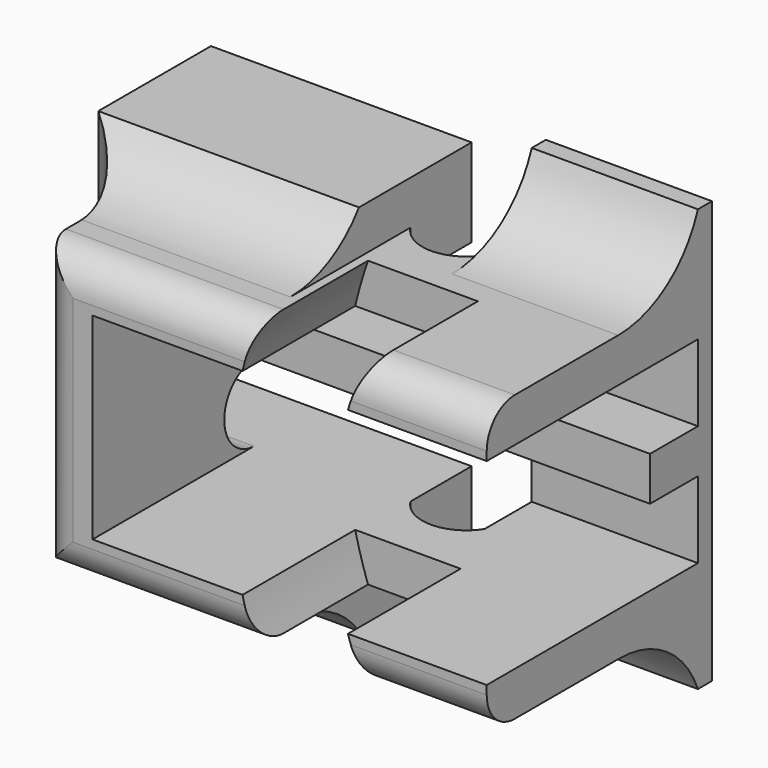
from build123d import *

# Parameters (mm, degrees)
F1_DEPTH      = 2.2
F2_DEPTH      = 4
F3_DEPTH      = 8
F5_W          = 4.721
F5_H          = 0.5
F6_DEPTH      = 2
F6_DEPTH_BACK = 10
F7_DEPTH      = 4
F8_T1_DEPTH   = 5.9270831351
F8_T3_DEPTH   = 8.1
F8_T5_DEPTH   = 4.721
F8_T11_DEPTH  = 12.0188296006
F8_T16_DEPTH  = 14.5648341529
F8_T24_DEPTH  = 14.5648341529
F8_T29_DEPTH  = 12.0188296006
F10_DEPTH     = 1.5
F12_DEPTH     = 2
F13_R         = 1


# Not quite as in the source:
# - a fillet or chamfer that OpenCascade refuses, or shapes differently, is made with other operations: its cross-section is extruded or revolved along the edge and cut away or added


with BuildPart() as f1:
    # F0 (on Front) → F1 (new body)
    with BuildSketch(Plane.XZ):
        with BuildLine():
            Line((-1.6440981598, 0.625), (-5.6, 0.625))
            Line((-5.6, 0.625), (-5.6, -0.625))
            Line((-5.6, -0.625), (-1.6440981598, -0.625))
            ThreePointArc((-1.6440981598, -0.625), (-1.6599999508, 0), (-1.6440981598, 0.625))
        make_face()
        with BuildLine():
            Line((-1.23, 0.625), (-1.6440981598, 0.625))
            ThreePointArc((-1.6440981598, 0.625), (-1.6599999508, 0), (-1.6440981598, -0.625))
            Line((-1.6440981598, -0.625), (-1.23, -0.625))
            Line((-1.23, -0.625), (1.2508001143, -0.625))
            ThreePointArc((1.2508001143, -0.625), (1.23, 0), (1.2508001143, 0.625))
            Line((1.2508001143, 0.625), (-1.23, 0.625))
        make_face()
        with BuildLine():
            Line((1.6420518568, 0.625), (1.2508001143, 0.625))
            ThreePointArc((1.2508001143, 0.625), (1.23, 0), (1.2508001143, -0.625))
            Line((1.2508001143, -0.625), (1.6420518568, -0.625))
            Line((1.6420518568, -0.625), (5.6, -0.625))
            Line((5.6, -0.625), (5.6, 0.625))
            Line((5.6, 0.625), (1.6420518568, 0.625))
        make_face()
    extrude(amount=F1_DEPTH)

    # F0 (on Front) → F2 (join)
    with BuildSketch(Plane.XZ):
        with BuildLine():
            Line((5.6, -2.8), (1.6566885771, -2.8))
            ThreePointArc((1.6566885771, -2.8), (1.8795878526, -3.4337692421), (2.1471830551, -4.05))
            Line((2.1471830551, -4.05), (5.6, -4.05))
            Line((5.6, -4.05), (5.6, -2.8))
        make_face()
        with BuildLine():
            Line((-1.23, -2.8), (-1.3368015602, -2.8))
            ThreePointArc((-1.3368015602, -2.8), (-1.1717307029, -3.4298126738), (-0.9735386938, -4.05))
            Line((-0.9735386938, -4.05), (0.8789681604, -4.05))
            Line((0.8789681604, -4.05), (2.1471830551, -4.05))
            ThreePointArc((2.1471830551, -4.05), (1.8795878526, -3.4337692421), (1.6566885771, -2.8))
            Line((1.6566885771, -2.8), (1.23, -2.8))
            Line((1.23, -2.8), (-1.23, -2.8))
        make_face()
        with BuildLine():
            Line((-1.735931594, -2.8), (-5.6, -2.8))
            Line((-5.6, -2.8), (-5.6, -4.05))
            Line((-5.6, -4.05), (-2.3307385194, -4.05))
            Line((-2.3307385194, -4.05), (-1.23, -4.05))
            Line((-1.23, -4.05), (-0.9735386938, -4.05))
            ThreePointArc((-0.9735386938, -4.05), (-1.1717307029, -3.4298126738), (-1.3368015602, -2.8))
            Line((-1.3368015602, -2.8), (-1.735931594, -2.8))
        make_face()
        Polygon((-7.1570831351, 4.05), (-5.6, 4.05), (-2.3307385194, 4.05), (-1.23, 4.05), (-1.23, 5.3), (-8.636245504, 5.3), (-8.636245504, -5.3), (-1.23, -5.3), (-1.23, -4.05), (-2.3307385194, -4.05), (-5.6, -4.05), (-7.1570831351, -4.05), align=None)
        Polygon((-5.6, -0.625), (-5.6, 0.625), (-5.6, 2.8), (-5.6, 4.05), (-7.1570831351, 4.05), (-7.1570831351, -4.05), (-5.6, -4.05), (-5.6, -2.8), align=None)
        with BuildLine():
            Line((-5.6, 4.05), (-5.6, 2.8))
            Line((-5.6, 2.8), (-1.735931594, 2.8))
            Line((-1.735931594, 2.8), (-1.3368015602, 2.8))
            ThreePointArc((-1.3368015602, 2.8), (-1.1717307029, 3.4298126738), (-0.9735386938, 4.05))
            Line((-0.9735386938, 4.05), (-1.23, 4.05))
            Line((-1.23, 4.05), (-2.3307385194, 4.05))
            Line((-2.3307385194, 4.05), (-5.6, 4.05))
        make_face()
        with BuildLine():
            ThreePointArc((-0.9735386938, 4.05), (-1.1717307029, 3.4298126738), (-1.3368015602, 2.8))
            Line((-1.3368015602, 2.8), (1.23, 2.8))
            Line((1.23, 2.8), (1.2939187969, 2.8))
            Line((1.2939187969, 2.8), (1.6566885771, 2.8))
            ThreePointArc((1.6566885771, 2.8), (1.8795878526, 3.4337692421), (2.1471830551, 4.05))
            Line((2.1471830551, 4.05), (0.8789681604, 4.05))
            Line((0.8789681604, 4.05), (-0.9735386938, 4.05))
        make_face()
        with BuildLine():
            ThreePointArc((2.1471830551, 4.05), (1.8795878526, 3.4337692421), (1.6566885771, 2.8))
            Line((1.6566885771, 2.8), (5.6, 2.8))
            Line((5.6, 2.8), (5.6, 4.05))
            Line((5.6, 4.05), (2.1471830551, 4.05))
        make_face()
    extrude(amount=F2_DEPTH)

    # F0 (on Front) → F3 (join)
    with BuildSketch(Plane.XZ):
        with BuildLine():
            ThreePointArc((2.1471830551, 4.05), (1.8795878526, 3.4337692421), (1.6566885771, 2.8))
            Line((1.6566885771, 2.8), (5.6, 2.8))
            Line((5.6, 2.8), (5.6, 4.05))
            Line((5.6, 4.05), (2.1471830551, 4.05))
        make_face()
        with BuildLine():
            Line((-5.6, 4.05), (-5.6, 2.8))
            Line((-5.6, 2.8), (-1.735931594, 2.8))
            Line((-1.735931594, 2.8), (-1.3368015602, 2.8))
            ThreePointArc((-1.3368015602, 2.8), (-1.1717307029, 3.4298126738), (-0.9735386938, 4.05))
            Line((-0.9735386938, 4.05), (-1.23, 4.05))
            Line((-1.23, 4.05), (-2.3307385194, 4.05))
            Line((-2.3307385194, 4.05), (-5.6, 4.05))
        make_face()
        Polygon((-5.6, -0.625), (-5.6, 0.625), (-5.6, 2.8), (-5.6, 4.05), (-7.1570831351, 4.05), (-7.1570831351, -4.05), (-5.6, -4.05), (-5.6, -2.8), align=None)
        with BuildLine():
            Line((-1.735931594, -2.8), (-5.6, -2.8))
            Line((-5.6, -2.8), (-5.6, -4.05))
            Line((-5.6, -4.05), (-2.3307385194, -4.05))
            Line((-2.3307385194, -4.05), (-1.23, -4.05))
            Line((-1.23, -4.05), (-0.9735386938, -4.05))
            ThreePointArc((-0.9735386938, -4.05), (-1.1717307029, -3.4298126738), (-1.3368015602, -2.8))
            Line((-1.3368015602, -2.8), (-1.735931594, -2.8))
        make_face()
        with BuildLine():
            Line((5.6, -2.8), (1.6566885771, -2.8))
            ThreePointArc((1.6566885771, -2.8), (1.8795878526, -3.4337692421), (2.1471830551, -4.05))
            Line((2.1471830551, -4.05), (5.6, -4.05))
            Line((5.6, -4.05), (5.6, -2.8))
        make_face()
    extrude(amount=F3_DEPTH)

    # F5 (on face) → F6 (join, two sides)
    with BuildSketch(Plane.XY.offset(4.05)) as f6_sk:
        with Locations((3.2395, -0.25)):
            Rectangle(F5_W, F5_H)
    extrude(amount=F6_DEPTH)
    extrude(f6_sk.sketch, amount=-F6_DEPTH_BACK)

    # F4 (on face) → F7 (cut)
    with BuildSketch(Plane(origin=(-8.636245504, 0, 0), x_dir=(0, -1, 0), z_dir=(-1, 0, 0))):
        with BuildLine():
            ThreePointArc((2.2, 0.625), (3.2875, 1.7125), (2.2, 2.8))
            Line((2.2, 2.8), (0, 2.8))
            Line((0, 2.8), (0, 0.625))
            Line((0, 0.625), (2.2, 0.625))
        make_face()
        with BuildLine():
            ThreePointArc((2.2659621103, -2.8), (3.3204810552, -1.6795189448), (2.2, -0.625))
            Line((2.2, -0.625), (0, -0.625))
            Line((0, -0.625), (0, -2.8))
            Line((0, -2.8), (2.2, -2.8))
            Line((2.2, -2.8), (2.2659621103, -2.8))
        make_face()
    extrude(amount=-F7_DEPTH, mode=Mode.SUBTRACT)

    # F8: fillet of radius 3 on 5 edges, made by hand

    # F8_s2 → F8_t1 (join)
    with BuildSketch(Plane.YZ.offset(-7.1570831351)):
        with BuildLine():
            ThreePointArc((-4, 5.3), (-5.0673921924, 4.380730437), (-6.4366985862, 4.05))
            Line((-6.4366985862, 4.05), (-4, 4.05))
            Line((-4, 4.05), (-4, 5.3))
        make_face()
        with BuildLine():
            ThreePointArc((-4, -5.3), (-5.0673921924, -4.380730437), (-6.4366985862, -4.05))
            Line((-6.4366985862, -4.05), (-4, -4.05))
            Line((-4, -4.05), (-4, -5.3))
        make_face()
    extrude(amount=F8_T1_DEPTH)

    # F8_s4 → F8_t3 (join)
    with BuildSketch(Plane.XY.offset(-4.05)):
        with BuildLine():
            ThreePointArc((-8.636245504, -4), (-7.5529985653, -5.0963889141), (-7.1570831351, -6.5859336612))
            Line((-7.1570831351, -6.5859336612), (-7.1570831351, -4))
            Line((-7.1570831351, -4), (-8.636245504, -4))
        make_face()
    extrude(amount=F8_T3_DEPTH)

    # F8_s6 → F8_t5 (join)
    with BuildSketch(Plane.YZ.offset(0.879)):
        with BuildLine():
            ThreePointArc((-0.5, -5.95), (-1.6028628458, -4.5700806465), (-3.2910571474, -4.05))
            Line((-3.2910571474, -4.05), (-0.5, -4.05))
            Line((-0.5, -4.05), (-0.5, -5.95))
        make_face()
        with BuildLine():
            ThreePointArc((-0.5, 6.05), (-1.5963763172, 4.6005102572), (-3.3284271247, 4.05))
            Line((-3.3284271247, 4.05), (-0.5, 4.05))
            Line((-0.5, 4.05), (-0.5, 6.05))
        make_face()
    extrude(amount=F8_T5_DEPTH)


with BuildPart() as f8_tool9:
    # F8_s10 → F8_t11 (new body)
    with BuildSketch(Plane.YZ.offset(-13.2488296006)):
        with BuildLine():
            ThreePointArc((-4, 5.3), (-5.0673921924, 4.380730437), (-6.4366985862, 4.05))
            Line((-6.4366985862, 4.05), (-4, 4.05))
            Line((-4, 4.05), (-4, 5.3))
        make_face()
    extrude(amount=F8_T11_DEPTH)

    split(bisect_by=Plane.YZ.offset(-7.1570831351), keep=Keep.BOTTOM)

    split(bisect_by=Plane.YZ.offset(-8.636245504), keep=Keep.TOP)


with BuildPart() as f8_tool14:
    # F8_s15 → F8_t16 (new body)
    with BuildSketch(Plane.XY.offset(-4.05)):
        with BuildLine():
            ThreePointArc((-8.636245504, -4), (-7.5529985653, -5.0963889141), (-7.1570831351, -6.5859336612))
            Line((-7.1570831351, -6.5859336612), (-7.1570831351, -4))
            Line((-7.1570831351, -4), (-8.636245504, -4))
        make_face()
    extrude(amount=F8_T16_DEPTH)

    split(bisect_by=Plane.XY.offset(5.3), keep=Keep.BOTTOM)

    split(bisect_by=Plane.XY.offset(4.05), keep=Keep.TOP)


with BuildPart() as f8_tool9_1:
    add(f8_tool9.part)

    # F8_t19: intersect F8_tool14
    add(f8_tool14.part, mode=Mode.INTERSECT)


with BuildPart() as f1_1:
    add(f1.part)

    # F8_t7: union F8_tool9
    add(f8_tool9_1.part)


with BuildPart() as f8_tool22:
    # F8_s23 → F8_t24 (new body)
    with BuildSketch(Plane.XY.offset(-10.5148341529)):
        with BuildLine():
            ThreePointArc((-8.636245504, -4), (-7.5529985653, -5.0963889141), (-7.1570831351, -6.5859336612))
            Line((-7.1570831351, -6.5859336612), (-7.1570831351, -4))
            Line((-7.1570831351, -4), (-8.636245504, -4))
        make_face()
    extrude(amount=F8_T24_DEPTH)

    split(bisect_by=Plane.XY.offset(-5.3), keep=Keep.TOP)

    split(bisect_by=Plane.XY.offset(-4.05), keep=Keep.BOTTOM)


with BuildPart() as f8_tool27:
    # F8_s28 → F8_t29 (new body)
    with BuildSketch(Plane.YZ.offset(-1.23)):
        with BuildLine():
            ThreePointArc((-4, -5.3), (-5.0673921924, -4.380730437), (-6.4366985862, -4.05))
            Line((-6.4366985862, -4.05), (-4, -4.05))
            Line((-4, -4.05), (-4, -5.3))
        make_face()
    extrude(amount=-F8_T29_DEPTH)

    split(bisect_by=Plane.YZ.offset(-7.1570831351), keep=Keep.BOTTOM)

    split(bisect_by=Plane.YZ.offset(-8.636245504), keep=Keep.TOP)


with BuildPart() as f8_tool22_1:
    add(f8_tool22.part)

    # F8_t32: intersect F8_tool27
    add(f8_tool27.part, mode=Mode.INTERSECT)


with BuildPart() as f1_2:
    add(f1_1.part)

    # F8_t20: union F8_tool22
    add(f8_tool22_1.part)

    # F9 (on face) → F10 (cut)
    with BuildSketch(Plane.XY.offset(4.05)):
        with BuildLine():
            Line((-1.23, 0), (-1.23, -2.1719092038))
            ThreePointArc((-1.23, -2.1719092038), (-0.1755, -2.7577127774), (0.879, -2.1719092038))
            Line((0.879, -2.1719092038), (0.879, 0))
            Line((0.879, 0), (-1.23, 0))
        make_face()
    extrude(amount=-F10_DEPTH, mode=Mode.SUBTRACT)

    # F11 (on face) → F12 (cut)
    with BuildSketch(Plane(origin=(0, 0, -4.05), x_dir=(1, 0, 0), z_dir=(0, 0, -1))):
        with BuildLine():
            ThreePointArc((0.879, 2.1719092038), (-0.1755, 2.7577127774), (-1.23, 2.1719092038))
            Line((-1.23, 2.1719092038), (-1.23, 0))
            Line((-1.23, 0), (0.879, 0))
            Line((0.879, 0), (0.879, 0.5))
            Line((0.879, 0.5), (0.879, 2.1719092038))
        make_face()
    extrude(amount=-F12_DEPTH, mode=Mode.SUBTRACT)

    # F13
    f13_edges = [f1_2.edges().sort_by_distance(p)[0] for p in [
        (-4.065311, -8, 4.05),
        (-7.157083, -8, 0),
        (-4.065311, -8, -4.05),
        (3.873592, -8, -4.05),
        (3.873592, -8, 4.05),
    ]]
    fillet(f13_edges, radius=F13_R)


solid = f1_2.part
